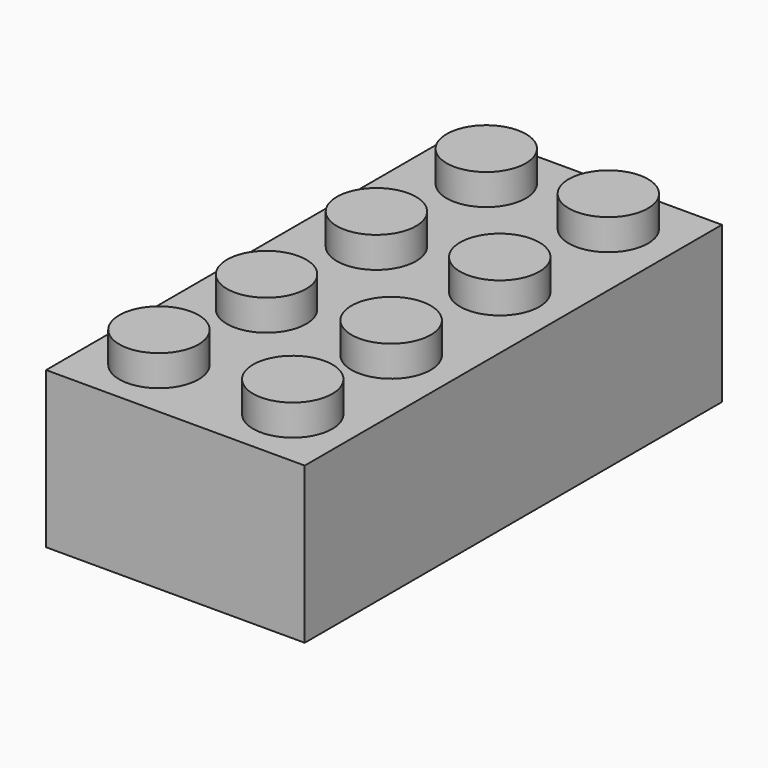
from build123d import *

# Parameters (mm, degrees)
F0_W      = 15.748
F0_H      = 9.4996
F1_DEPTH  = 31.75
F2_R      = 2.413
F4_DEPTH  = 1.8796
F3_R      = 2.413
F5_DEPTH  = 1.8796
F6_T      = -1.2192
F7_R      = 3.175
F8_DEPTH  = 7.3152
F9_DEPTH  = 7.3152
F10_DEPTH = 7.3152
F12_DEPTH = 6.7881


with BuildPart() as f1:
    # F0 (on Front) → F1 (new body)
    with BuildSketch(Plane.XZ):
        with Locations((-0.199874863, 0.3277875761)):
            Rectangle(F0_W, F0_H)
    extrude(amount=F1_DEPTH)

    # F2 (on face) → F4 (join)
    with BuildSketch(Plane.XY.offset(5.0775875761)):
        with Locations((-4.2189443147, -27.9770765305)):
            Circle(F2_R)
        with Locations((3.9266556272, -27.978049837)):
            Circle(F2_R)
    extrude(amount=F4_DEPTH)

    # F3 (on face) → F5 (join)
    with BuildSketch(Plane.XY.offset(5.0775875761)):
        with Locations((3.7918896414, -20.3214651638)):
            Circle(F3_R)
        with Locations((3.75443, -12.0085638718)):
            Circle(F3_R)
        with Locations((3.7169703586, -3.6956625797)):
            Circle(F3_R)
        with Locations((-3.7169703586, -3.6956625797)):
            Circle(F3_R)
        with Locations((-3.75443, -12.0085638718)):
            Circle(F3_R)
        with Locations((-3.7918896414, -20.3214651638)):
            Circle(F3_R)
    extrude(amount=F5_DEPTH)

    # F6
    f6_openings = [f1.faces().sort_by_distance(p)[0] for p in [
        (-0.199875, -15.875, -4.422012),
    ]]
    offset(amount=F6_T, openings=f6_openings, kind=Kind.INTERSECTION)

    # F7 (on face) → F8 (join)
    with BuildSketch(Plane(origin=(0, 0, 3.8583875761), x_dir=(1, 0, 0), z_dir=(0, 0, -1))):
        with Locations((0, 8.1207330356)):
            Circle(F7_R)
    extrude(amount=F8_DEPTH)

    # F7 (on face) → F9 (join)
    with BuildSketch(Plane(origin=(0, 0, 3.8583875761), x_dir=(1, 0, 0), z_dir=(0, 0, -1))):
        with Locations((0, 25.0235652365)):
            Circle(F7_R)
    extrude(amount=F9_DEPTH)

    # F7 (on face) → F10 (join)
    with BuildSketch(Plane(origin=(0, 0, 3.8583875761), x_dir=(1, 0, 0), z_dir=(0, 0, -1))):
        with BuildLine():
            ThreePointArc((-3.175, 16.6939621039), (0, 13.5189621039), (3.175, 16.6939621039))
            ThreePointArc((3.175, 16.6939621039), (0, 19.8689621039), (-3.175, 16.6939621039))
        make_face()
    extrude(amount=F10_DEPTH)

    # F11 (on face) → F12 (join)
    with BuildSketch(Plane(origin=(0, 0, 3.8583875761), x_dir=(1, 0, 0), z_dir=(0, 0, -1))):
        with BuildLine():
            ThreePointArc((-3.1611326952, 16.3975416535), (-3.1749888394, 16.7023805357), (-3.1595163506, 17.0071416535))
            Line((-3.1595163506, 17.0071416535), (-6.854674863, 17.0071416535))
            Line((-6.854674863, 17.0071416535), (-6.854674863, 16.3975416535))
            Line((-6.854674863, 16.3975416535), (-3.1611326952, 16.3975416535))
        make_face()
        with BuildLine():
            Line((6.454925137, 17.0071416535), (3.1595163506, 17.0071416535))
            ThreePointArc((3.1595163506, 17.0071416535), (3.1711267251, 16.8507431404), (3.175, 16.6939621039))
            ThreePointArc((3.175, 16.6939621039), (3.171531279, 16.5455897804), (3.1611326952, 16.3975416535))
            Line((3.1611326952, 16.3975416535), (6.454925137, 16.3975416535))
            Line((6.454925137, 16.3975416535), (6.454925137, 17.0071416535))
        make_face()
    extrude(amount=F12_DEPTH)


solid = f1.part
